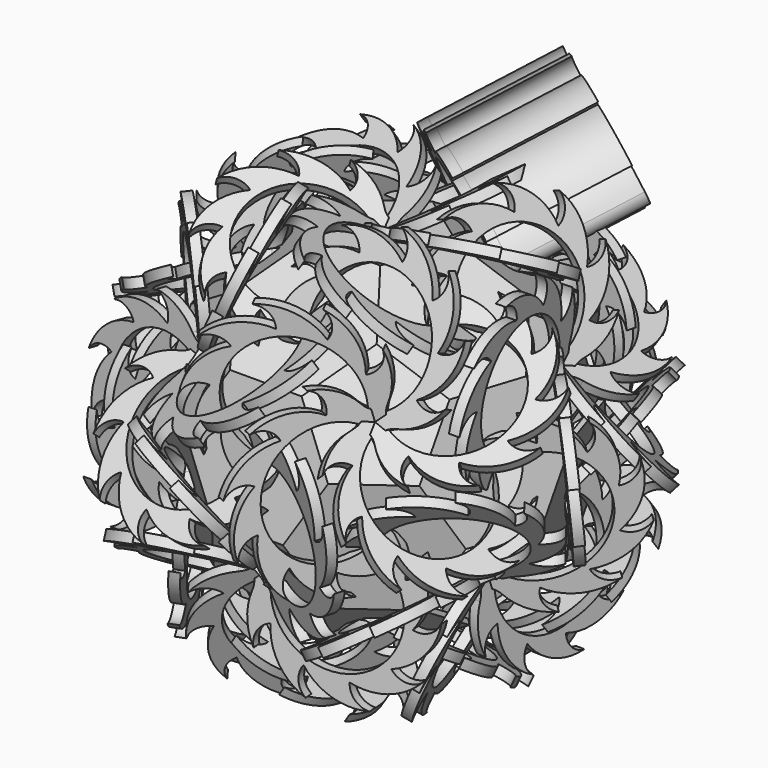
from build123d import *

# Parameters (mm, degrees)
F2_DEPTH  = 1
F3_DEPTH  = 1
F4_ANGLE  = -37.377368
F6_COUNT  = 5
F6_ANGLE  = 288
F9_DEPTH  = 2
F10_R     = 5
F12_ANGLE = 65
F13_COUNT = 5
F13_ANGLE = 288
F15_COUNT = 3
F15_ANGLE = 240
F16_COUNT = 5
F16_ANGLE = 288
F17_COUNT = 2
F17_ANGLE = 120
F18_COUNT = 3
F18_ANGLE = 240
F22_COUNT = 3
F22_ANGLE = 144
F26_COUNT = 3
F26_ANGLE = 144
F29_COUNT = 2
F29_ANGLE = 120
F32_COUNT = 3
F32_ANGLE = 144
F36_COUNT = 3
F36_ANGLE = 240
F40_COUNT = 3
F40_ANGLE = 144
F44_COUNT = 3
F44_ANGLE = 144
F48_COUNT = 2
F48_ANGLE = 120
F52_COUNT = 2
F52_ANGLE = 120
F56_COUNT = 2
F56_ANGLE = 120
F60_COUNT = 2
F60_ANGLE = 120
F66_DEPTH = 25


with BuildPart() as f2:
    # F0 (on Top) → F2 (new body)
    with BuildSketch(Plane.XY):
        Polygon((0, -10.3228644035), (7.5, -10.3228644035), (12.1352549156, 3.9429833409), (0, 12.7597621253), align=None)
        Polygon((-7.5, -10.3228644035), (0, -10.3228644035), (0, 12.7597621253), (-12.1352549156, 3.9429833409), align=None)
    extrude(amount=-F2_DEPTH)


with BuildPart() as f3:
    # F1 (on Top) → F3 (new body)
    with BuildSketch(Plane.XY):
        Polygon((32.2091731064, -18.3513614234), (36.844428022, -4.085513679), (26.8074689266, 7.0616587032), (12.1352549156, 3.9429833409), (7.5, -10.3228644035), (17.5369590954, -21.4700367857), align=None)
    extrude(amount=-F3_DEPTH)


with BuildPart() as f3_1:
    # F4: moved
    add(f3.part.rotate(Axis((9.8176274578, -3.1899405313, 0), (-0.3090169944, -0.9510565163, 0)), F4_ANGLE))


with BuildPart() as f6_1:
    # F6: instance of F3
    add(f3_1.part.rotate(Axis((0, 0, 3.8664315362), (0, 0, 1)), 1 * F6_ANGLE / (F6_COUNT - 1)))


with BuildPart() as f6_2:
    # F6: instance of F3
    add(f3_1.part.rotate(Axis((0, 0, 3.8664315362), (0, 0, 1)), 2 * F6_ANGLE / (F6_COUNT - 1)))


with BuildPart() as f6_3:
    # F6: instance of F3
    add(f3_1.part.rotate(Axis((0, 0, 3.8664315362), (0, 0, 1)), 3 * F6_ANGLE / (F6_COUNT - 1)))


with BuildPart() as f6_4:
    # F6: instance of F3
    add(f3_1.part.rotate(Axis((0, 0, 3.8664315362), (0, 0, 1)), 4 * F6_ANGLE / (F6_COUNT - 1)))


with BuildPart() as f9:
    # F8 (on Right) → F9 (new body)
    with BuildSketch(Plane.YZ):
        with BuildLine():
            ThreePointArc((-20.0381562793, -7.4218225341), (-18.0432138806, 14.7456768661), (-1.371596125, 0))
            ThreePointArc((-1.371596125, 0), (1.2710572909, -2.1110060804), (1.0658705895, 1.265065922))
            ThreePointArc((1.0658705895, 1.265065922), (3.462744203, 7.3677169674), (2.5001799222, 13.8531485572))
            ThreePointArc((2.5001799222, 13.8531485572), (1.8396441745, 10.7438611605), (-0.8004298525, 8.9735547684))
            ThreePointArc((-0.8004298525, 8.9735547684), (-2.1304901639, 15.9377846017), (-6.983453041, 21.1067602176))
            ThreePointArc((-6.983453041, 21.1067602176), (-5.7243130519, 18.2607184854), (-6.7542303289, 15.3239417734))
            ThreePointArc((-6.7542303289, 15.3239417734), (-11.923743314, 20.1763322255), (-18.8881203911, 21.5056213332))
            ThreePointArc((-18.8881203911, 21.5056213332), (-16.196593384, 19.9432291213), (-15.3036199233, 16.9619566661))
            ThreePointArc((-15.3036199233, 16.9619566661), (-22.3380073271, 17.8490595111), (-28.7536432712, 14.8309188523))
            ThreePointArc((-28.7536432712, 14.8309188523), (-25.6578010812, 15.1489568819), (-23.1830223937, 13.2619334316))
            ThreePointArc((-23.1830223937, 13.2619334316), (-29.3953873179, 9.8449055341), (-32.8117272579, 3.6321622578))
            ThreePointArc((-32.8117272579, 3.6321622578), (-30.4940763777, 5.7091508113), (-27.3827738075, 5.6371551864))
            ThreePointArc((-27.3827738075, 5.6371551864), (-30.4002040016, -0.7788149372), (-29.5123221974, -7.813104063))
            ThreePointArc((-29.5123221974, -7.813104063), (-28.8581264893, -4.7705040188), (-26.2987118688, -2.9999719366))
            ThreePointArc((-26.2987118688, -2.9999719366), (-26.0274642787, -7.0575500385), (-24.4889350399, -10.821914937))
            ThreePointArc((-24.4889350399, -10.821914937), (-20.5634994581, -11.3472581158), (-20.0381562793, -7.4218225341))
        make_face()
    extrude(amount=-F9_DEPTH)

    # F10
    f10_edges = [f9.edges().sort_by_distance(p)[0] for p in [
        (-1, 1.065871, 1.265066),
    ]]
    fillet(f10_edges, radius=F10_R)


with BuildPart() as f9_1:
    # F12: moved
    add(f9.part.rotate(Axis((0, -10.3228644132, -3.9429833282), (0, -0.9341723595, -0.3568220885)), F12_ANGLE))


with BuildPart() as f13_1:
    # F13: instance of F9
    add(f9_1.part.rotate(Axis((0, 0, 14.2103461549), (0, 0, 1)), 1 * F13_ANGLE / (F13_COUNT - 1)))


with BuildPart() as f13_2:
    # F13: instance of F9
    add(f9_1.part.rotate(Axis((0, 0, 14.2103461549), (0, 0, 1)), 2 * F13_ANGLE / (F13_COUNT - 1)))


with BuildPart() as f13_3:
    # F13: instance of F9
    add(f9_1.part.rotate(Axis((0, 0, 14.2103461549), (0, 0, 1)), 3 * F13_ANGLE / (F13_COUNT - 1)))


with BuildPart() as f13_4:
    # F13: instance of F9
    add(f9_1.part.rotate(Axis((0, 0, 14.2103461549), (0, 0, 1)), 4 * F13_ANGLE / (F13_COUNT - 1)))


with BuildPart() as f15_1:
    # F15: instance of F9
    add(f9_1.part.rotate(Axis((0, -25.3455492518, -1.7338218178), (0, -0.6070619963, 0.7946544738)), 1 * F15_ANGLE / (F15_COUNT - 1)))


with BuildPart() as f15_2:
    # F15: instance of F9
    add(f9_1.part.rotate(Axis((0, -25.3455492518, -1.7338218178), (0, -0.6070619963, 0.7946544738)), 2 * F15_ANGLE / (F15_COUNT - 1)))


with BuildPart() as f16_1:
    # F16: instance of F15_2
    add(f15_2.part.rotate(Axis((0, 0, 14.2103461549), (0, 0, 1)), 1 * F16_ANGLE / (F16_COUNT - 1)))


with BuildPart() as f16_2:
    # F16: instance of F15_2
    add(f15_2.part.rotate(Axis((0, 0, 14.2103461549), (0, 0, 1)), 2 * F16_ANGLE / (F16_COUNT - 1)))


with BuildPart() as f16_3:
    # F16: instance of F15_2
    add(f15_2.part.rotate(Axis((0, 0, 14.2103461549), (0, 0, 1)), 3 * F16_ANGLE / (F16_COUNT - 1)))


with BuildPart() as f16_4:
    # F16: instance of F15_2
    add(f15_2.part.rotate(Axis((0, 0, 14.2103461549), (0, 0, 1)), 4 * F16_ANGLE / (F16_COUNT - 1)))


with BuildPart() as f16_5:
    # F16: instance of F15_1
    add(f15_1.part.rotate(Axis((0, 0, 14.2103461549), (0, 0, 1)), 1 * F16_ANGLE / (F16_COUNT - 1)))


with BuildPart() as f16_6:
    # F16: instance of F15_1
    add(f15_1.part.rotate(Axis((0, 0, 14.2103461549), (0, 0, 1)), 2 * F16_ANGLE / (F16_COUNT - 1)))


with BuildPart() as f16_7:
    # F16: instance of F15_1
    add(f15_1.part.rotate(Axis((0, 0, 14.2103461549), (0, 0, 1)), 3 * F16_ANGLE / (F16_COUNT - 1)))


with BuildPart() as f16_8:
    # F16: instance of F15_1
    add(f15_1.part.rotate(Axis((0, 0, 14.2103461549), (0, 0, 1)), 4 * F16_ANGLE / (F16_COUNT - 1)))


with BuildPart() as f17_1:
    # F17: instance of F3
    add(f3_1.part.rotate(Axis((0, -25.3455492518, -1.7338218178), (0, 0.6070619963, -0.7946544738)), 1 * F17_ANGLE / (F17_COUNT - 1)))


with BuildPart() as f17_2:
    # F17: instance of F16_5
    add(f16_5.part.rotate(Axis((0, -25.3455492518, -1.7338218178), (0, 0.6070619963, -0.7946544738)), 1 * F17_ANGLE / (F17_COUNT - 1)))


with BuildPart() as f17_3:
    # F17: instance of F13_1
    add(f13_1.part.rotate(Axis((0, -25.3455492518, -1.7338218178), (0, 0.6070619963, -0.7946544738)), 1 * F17_ANGLE / (F17_COUNT - 1)))


with BuildPart() as f17_4:
    # F17: instance of F16_1
    add(f16_1.part.rotate(Axis((0, -25.3455492518, -1.7338218178), (0, 0.6070619963, -0.7946544738)), 1 * F17_ANGLE / (F17_COUNT - 1)))


with BuildPart() as f18_1:
    # F18: instance of F2
    add(f2.part.rotate(Axis((0, -25.3455492518, -1.7338218178), (0, -0.6070619963, 0.7946544738)), 1 * F18_ANGLE / (F18_COUNT - 1)))


with BuildPart() as f18_2:
    # F18: instance of F2
    add(f2.part.rotate(Axis((0, -25.3455492518, -1.7338218178), (0, -0.6070619963, 0.7946544738)), 2 * F18_ANGLE / (F18_COUNT - 1)))


with BuildPart() as f18_3:
    # F18: instance of F13_2
    add(f13_2.part.rotate(Axis((0, -25.3455492518, -1.7338218178), (0, -0.6070619963, 0.7946544738)), 1 * F18_ANGLE / (F18_COUNT - 1)))


with BuildPart() as f18_4:
    # F18: instance of F13_2
    add(f13_2.part.rotate(Axis((0, -25.3455492518, -1.7338218178), (0, -0.6070619963, 0.7946544738)), 2 * F18_ANGLE / (F18_COUNT - 1)))


with BuildPart() as f18_5:
    # F18: instance of F13_3
    add(f13_3.part.rotate(Axis((0, -25.3455492518, -1.7338218178), (0, -0.6070619963, 0.7946544738)), 1 * F18_ANGLE / (F18_COUNT - 1)))


with BuildPart() as f18_6:
    # F18: instance of F13_3
    add(f13_3.part.rotate(Axis((0, -25.3455492518, -1.7338218178), (0, -0.6070619963, 0.7946544738)), 2 * F18_ANGLE / (F18_COUNT - 1)))


with BuildPart() as f22_1:
    # F22: instance of F17_1
    add(f17_1.part.rotate(Axis((-18.9711930891, -26.1116072266, -18.7737157723), (0.5257311104, 0.7236067968, -0.4472135991)), 1 * F22_ANGLE / (F22_COUNT - 1)))


with BuildPart() as f22_2:
    # F22: instance of F17_1
    add(f17_1.part.rotate(Axis((-18.9711930891, -26.1116072266, -18.7737157723), (0.5257311104, 0.7236067968, -0.4472135991)), 2 * F22_ANGLE / (F22_COUNT - 1)))


with BuildPart() as f22_3:
    # F22: instance of F17_3
    add(f17_3.part.rotate(Axis((-18.9711930891, -26.1116072266, -18.7737157723), (0.5257311104, 0.7236067968, -0.4472135991)), 1 * F22_ANGLE / (F22_COUNT - 1)))


with BuildPart() as f22_4:
    # F22: instance of F17_3
    add(f17_3.part.rotate(Axis((-18.9711930891, -26.1116072266, -18.7737157723), (0.5257311104, 0.7236067968, -0.4472135991)), 2 * F22_ANGLE / (F22_COUNT - 1)))


with BuildPart() as f22_5:
    # F22: instance of F17_4
    add(f17_4.part.rotate(Axis((-18.9711930891, -26.1116072266, -18.7737157723), (0.5257311104, 0.7236067968, -0.4472135991)), 1 * F22_ANGLE / (F22_COUNT - 1)))


with BuildPart() as f22_6:
    # F22: instance of F17_4
    add(f17_4.part.rotate(Axis((-18.9711930891, -26.1116072266, -18.7737157723), (0.5257311104, 0.7236067968, -0.4472135991)), 2 * F22_ANGLE / (F22_COUNT - 1)))


with BuildPart() as f22_7:
    # F22: instance of F17_2
    add(f17_2.part.rotate(Axis((-18.9711930891, -26.1116072266, -18.7737157723), (0.5257311104, 0.7236067968, -0.4472135991)), 1 * F22_ANGLE / (F22_COUNT - 1)))


with BuildPart() as f22_8:
    # F22: instance of F17_2
    add(f17_2.part.rotate(Axis((-18.9711930891, -26.1116072266, -18.7737157723), (0.5257311104, 0.7236067968, -0.4472135991)), 2 * F22_ANGLE / (F22_COUNT - 1)))


with BuildPart() as f26_1:
    # F26: instance of F3
    add(f3_1.part.rotate(Axis((20.2758098134, -27.9072581024, -17.6639424888), (-0.5257311104, 0.7236067968, -0.4472135991)), 1 * F26_ANGLE / (F26_COUNT - 1)))


with BuildPart() as f26_2:
    # F26: instance of F3
    add(f3_1.part.rotate(Axis((20.2758098134, -27.9072581024, -17.6639424888), (-0.5257311104, 0.7236067968, -0.4472135991)), 2 * F26_ANGLE / (F26_COUNT - 1)))


with BuildPart() as f26_3:
    # F26: instance of F16_1
    add(f16_1.part.rotate(Axis((20.2758098134, -27.9072581024, -17.6639424888), (-0.5257311104, 0.7236067968, -0.4472135991)), 1 * F26_ANGLE / (F26_COUNT - 1)))


with BuildPart() as f26_4:
    # F26: instance of F16_1
    add(f16_1.part.rotate(Axis((20.2758098134, -27.9072581024, -17.6639424888), (-0.5257311104, 0.7236067968, -0.4472135991)), 2 * F26_ANGLE / (F26_COUNT - 1)))


with BuildPart() as f26_5:
    # F26: instance of F13_1
    add(f13_1.part.rotate(Axis((20.2758098134, -27.9072581024, -17.6639424888), (-0.5257311104, 0.7236067968, -0.4472135991)), 1 * F26_ANGLE / (F26_COUNT - 1)))


with BuildPart() as f26_6:
    # F26: instance of F13_1
    add(f13_1.part.rotate(Axis((20.2758098134, -27.9072581024, -17.6639424888), (-0.5257311104, 0.7236067968, -0.4472135991)), 2 * F26_ANGLE / (F26_COUNT - 1)))


with BuildPart() as f26_7:
    # F26: instance of F16_5
    add(f16_5.part.rotate(Axis((20.2758098134, -27.9072581024, -17.6639424888), (-0.5257311104, 0.7236067968, -0.4472135991)), 1 * F26_ANGLE / (F26_COUNT - 1)))


with BuildPart() as f26_8:
    # F26: instance of F16_5
    add(f16_5.part.rotate(Axis((20.2758098134, -27.9072581024, -17.6639424888), (-0.5257311104, 0.7236067968, -0.4472135991)), 2 * F26_ANGLE / (F26_COUNT - 1)))


with BuildPart() as f29_1:
    # F29: instance of F18_2
    add(f18_2.part.rotate(Axis((0, -40.5030693029, -27.1761785704), (0, 0.9822469455, -0.1875924789)), 1 * F29_ANGLE / (F29_COUNT - 1)))


with BuildPart() as f32_1:
    # F32: instance of F26_2
    add(f26_2.part.rotate(Axis((0, -41.1465715097, -55.4848620892), (0, 0.8944271941, 0.4472135893)), 1 * F32_ANGLE / (F32_COUNT - 1)))


with BuildPart() as f32_2:
    # F32: instance of F26_2
    add(f26_2.part.rotate(Axis((0, -41.1465715097, -55.4848620892), (0, 0.8944271941, 0.4472135893)), 2 * F32_ANGLE / (F32_COUNT - 1)))


with BuildPart() as f32_3:
    # F32: instance of F26_4
    add(f26_4.part.rotate(Axis((0, -41.1465715097, -55.4848620892), (0, 0.8944271941, 0.4472135893)), 1 * F32_ANGLE / (F32_COUNT - 1)))


with BuildPart() as f32_4:
    # F32: instance of F26_4
    add(f26_4.part.rotate(Axis((0, -41.1465715097, -55.4848620892), (0, 0.8944271941, 0.4472135893)), 2 * F32_ANGLE / (F32_COUNT - 1)))


with BuildPart() as f32_5:
    # F32: instance of F26_6
    add(f26_6.part.rotate(Axis((0, -41.1465715097, -55.4848620892), (0, 0.8944271941, 0.4472135893)), 1 * F32_ANGLE / (F32_COUNT - 1)))


with BuildPart() as f32_6:
    # F32: instance of F26_6
    add(f26_6.part.rotate(Axis((0, -41.1465715097, -55.4848620892), (0, 0.8944271941, 0.4472135893)), 2 * F32_ANGLE / (F32_COUNT - 1)))


with BuildPart() as f32_7:
    # F32: instance of F18_4
    add(f18_4.part.rotate(Axis((0, -41.1465715097, -55.4848620892), (0, 0.8944271941, 0.4472135893)), 1 * F32_ANGLE / (F32_COUNT - 1)))


with BuildPart() as f32_8:
    # F32: instance of F18_4
    add(f18_4.part.rotate(Axis((0, -41.1465715097, -55.4848620892), (0, 0.8944271941, 0.4472135893)), 2 * F32_ANGLE / (F32_COUNT - 1)))


with BuildPart() as f36_1:
    # F36: instance of F2
    add(f2.part.rotate(Axis((-17.4030966331, 23.953307566, 3.8456892929), (0.3568220886, -0.4911234716, -0.7946544738)), 1 * F36_ANGLE / (F36_COUNT - 1)))


with BuildPart() as f36_2:
    # F36: instance of F2
    add(f2.part.rotate(Axis((-17.4030966331, 23.953307566, 3.8456892929), (0.3568220886, -0.4911234716, -0.7946544738)), 2 * F36_ANGLE / (F36_COUNT - 1)))


with BuildPart() as f40_1:
    # F40: instance of F22_2
    add(f22_2.part.rotate(Axis((-43.9943598437, 14.2946340797, -11.7823727251), (0.8506508064, -0.2763932025, -0.4472135991)), 1 * F40_ANGLE / (F40_COUNT - 1)))


with BuildPart() as f40_2:
    # F40: instance of F22_2
    add(f22_2.part.rotate(Axis((-43.9943598437, 14.2946340797, -11.7823727251), (0.8506508064, -0.2763932025, -0.4472135991)), 2 * F40_ANGLE / (F40_COUNT - 1)))


with BuildPart() as f40_3:
    # F40: instance of F22_6
    add(f22_6.part.rotate(Axis((-43.9943598437, 14.2946340797, -11.7823727251), (0.8506508064, -0.2763932025, -0.4472135991)), 1 * F40_ANGLE / (F40_COUNT - 1)))


with BuildPart() as f40_4:
    # F40: instance of F22_6
    add(f22_6.part.rotate(Axis((-43.9943598437, 14.2946340797, -11.7823727251), (0.8506508064, -0.2763932025, -0.4472135991)), 2 * F40_ANGLE / (F40_COUNT - 1)))


with BuildPart() as f40_5:
    # F40: instance of F22_4
    add(f22_4.part.rotate(Axis((-43.9943598437, 14.2946340797, -11.7823727251), (0.8506508064, -0.2763932025, -0.4472135991)), 1 * F40_ANGLE / (F40_COUNT - 1)))


with BuildPart() as f40_6:
    # F40: instance of F22_4
    add(f22_4.part.rotate(Axis((-43.9943598437, 14.2946340797, -11.7823727251), (0.8506508064, -0.2763932025, -0.4472135991)), 2 * F40_ANGLE / (F40_COUNT - 1)))


with BuildPart() as f40_7:
    # F40: instance of F18_3
    add(f18_3.part.rotate(Axis((-43.9943598437, 14.2946340797, -11.7823727251), (0.8506508064, -0.2763932025, -0.4472135991)), 1 * F40_ANGLE / (F40_COUNT - 1)))


with BuildPart() as f40_8:
    # F40: instance of F18_3
    add(f18_3.part.rotate(Axis((-43.9943598437, 14.2946340797, -11.7823727251), (0.8506508064, -0.2763932025, -0.4472135991)), 2 * F40_ANGLE / (F40_COUNT - 1)))


with BuildPart() as f44_1:
    # F44: instance of F40_2
    add(f40_2.part.rotate(Axis((1.534e-07, 54.8190866503, -7.5020330917), (-6.9e-09, -0.8944271892, -0.4472135991)), 1 * F44_ANGLE / (F44_COUNT - 1)))


with BuildPart() as f44_2:
    # F44: instance of F40_2
    add(f40_2.part.rotate(Axis((1.534e-07, 54.8190866503, -7.5020330917), (-6.9e-09, -0.8944271892, -0.4472135991)), 2 * F44_ANGLE / (F44_COUNT - 1)))


with BuildPart() as f44_3:
    # F44: instance of F40_6
    add(f40_6.part.rotate(Axis((1.534e-07, 54.8190866503, -7.5020330917), (-6.9e-09, -0.8944271892, -0.4472135991)), 1 * F44_ANGLE / (F44_COUNT - 1)))


with BuildPart() as f44_4:
    # F44: instance of F40_6
    add(f40_6.part.rotate(Axis((1.534e-07, 54.8190866503, -7.5020330917), (-6.9e-09, -0.8944271892, -0.4472135991)), 2 * F44_ANGLE / (F44_COUNT - 1)))


with BuildPart() as f44_5:
    # F44: instance of F40_8
    add(f40_8.part.rotate(Axis((1.534e-07, 54.8190866503, -7.5020330917), (-6.9e-09, -0.8944271892, -0.4472135991)), 1 * F44_ANGLE / (F44_COUNT - 1)))


with BuildPart() as f44_6:
    # F44: instance of F40_8
    add(f40_8.part.rotate(Axis((1.534e-07, 54.8190866503, -7.5020330917), (-6.9e-09, -0.8944271892, -0.4472135991)), 2 * F44_ANGLE / (F44_COUNT - 1)))


with BuildPart() as f44_7:
    # F44: instance of F40_4
    add(f40_4.part.rotate(Axis((1.534e-07, 54.8190866503, -7.5020330917), (-6.9e-09, -0.8944271892, -0.4472135991)), 1 * F44_ANGLE / (F44_COUNT - 1)))


with BuildPart() as f44_8:
    # F44: instance of F40_4
    add(f40_4.part.rotate(Axis((1.534e-07, 54.8190866503, -7.5020330917), (-6.9e-09, -0.8944271892, -0.4472135991)), 2 * F44_ANGLE / (F44_COUNT - 1)))


with BuildPart() as f48_1:
    # F48: instance of F22_2
    add(f22_2.part.rotate(Axis((-45.320051719, 14.7253777202, -44.0123603845), (0.9341723533, -0.3035310175, 0.1875924726)), 1 * F48_ANGLE / (F48_COUNT - 1)))


with BuildPart() as f48_2:
    # F48: instance of F22_4
    add(f22_4.part.rotate(Axis((-45.320051719, 14.7253777202, -44.0123603845), (0.9341723533, -0.3035310175, 0.1875924726)), 1 * F48_ANGLE / (F48_COUNT - 1)))


with BuildPart() as f48_3:
    # F48: instance of F22_6
    add(f22_6.part.rotate(Axis((-45.320051719, 14.7253777202, -44.0123603845), (0.9341723533, -0.3035310175, 0.1875924726)), 1 * F48_ANGLE / (F48_COUNT - 1)))


with BuildPart() as f48_4:
    # F48: instance of F18_3
    add(f18_3.part.rotate(Axis((-45.320051719, 14.7253777202, -44.0123603845), (0.9341723533, -0.3035310175, 0.1875924726)), 1 * F48_ANGLE / (F48_COUNT - 1)))


with BuildPart() as f52_1:
    # F52: instance of F16_5
    add(f16_5.part.rotate(Axis((51.1630279448, -16.6238756598, -24.6374564773), (-0.9341723577, 0.3035310035, -0.1875924733)), 1 * F52_ANGLE / (F52_COUNT - 1)))


with BuildPart() as f52_2:
    # F52: instance of F13_1
    add(f13_1.part.rotate(Axis((51.1630279448, -16.6238756598, -24.6374564773), (-0.9341723577, 0.3035310035, -0.1875924733)), 1 * F52_ANGLE / (F52_COUNT - 1)))


with BuildPart() as f52_3:
    # F52: instance of F16_1
    add(f16_1.part.rotate(Axis((51.1630279448, -16.6238756598, -24.6374564773), (-0.9341723577, 0.3035310035, -0.1875924733)), 1 * F52_ANGLE / (F52_COUNT - 1)))


with BuildPart() as f52_4:
    # F52: instance of F3
    add(f3_1.part.rotate(Axis((51.1630279448, -16.6238756598, -24.6374564773), (-0.9341723577, 0.3035310035, -0.1875924733)), 1 * F52_ANGLE / (F52_COUNT - 1)))


with BuildPart() as f56_1:
    # F56: instance of F26_2
    add(f26_2.part.rotate(Axis((20.2389789509, -27.8565650407, -79.9844450272), (-0.3568220897, 0.4911234788, 0.7946544689)), 1 * F56_ANGLE / (F56_COUNT - 1)))


with BuildPart() as f56_2:
    # F56: instance of F26_4
    add(f26_4.part.rotate(Axis((20.2389789509, -27.8565650407, -79.9844450272), (-0.3568220897, 0.4911234788, 0.7946544689)), 1 * F56_ANGLE / (F56_COUNT - 1)))


with BuildPart() as f56_3:
    # F56: instance of F26_6
    add(f26_6.part.rotate(Axis((20.2389789509, -27.8565650407, -79.9844450272), (-0.3568220897, 0.4911234788, 0.7946544689)), 1 * F56_ANGLE / (F56_COUNT - 1)))


with BuildPart() as f56_4:
    # F56: instance of F18_4
    add(f18_4.part.rotate(Axis((20.2389789509, -27.8565650407, -79.9844450272), (-0.3568220897, 0.4911234788, 0.7946544689)), 1 * F56_ANGLE / (F56_COUNT - 1)))


with BuildPart() as f60_1:
    # F60: instance of F52_4
    add(f52_4.part.rotate(Axis((24.2012826257, 7.8634731584, -68.221784607), (-0.5773502692, -0.1875924683, 0.7946544737)), 1 * F60_ANGLE / (F60_COUNT - 1)))


with BuildPart() as f60_2:
    # F60: instance of F52_3
    add(f52_3.part.rotate(Axis((24.2012826257, 7.8634731584, -68.221784607), (-0.5773502692, -0.1875924683, 0.7946544737)), 1 * F60_ANGLE / (F60_COUNT - 1)))


with BuildPart() as f60_3:
    # F60: instance of F52_1
    add(f52_1.part.rotate(Axis((24.2012826257, 7.8634731584, -68.221784607), (-0.5773502692, -0.1875924683, 0.7946544737)), 1 * F60_ANGLE / (F60_COUNT - 1)))


with BuildPart() as f60_4:
    # F60: instance of F52_2
    add(f52_2.part.rotate(Axis((24.2012826257, 7.8634731584, -68.221784607), (-0.5773502692, -0.1875924683, 0.7946544737)), 1 * F60_ANGLE / (F60_COUNT - 1)))


with BuildPart() as f66:
    # F66 (new): a face of the model
    f66_faces = [f16_2.part.faces().sort_by_distance(p)[0] for p in [
        (1.31810176, 30.9628284564, -20.5883774051),
    ]]
    extrude(f66_faces, amount=F66_DEPTH)


solid = Compound([f2.part, f3_1.part, f6_1.part, f6_2.part, f6_3.part, f6_4.part, f9_1.part, f13_1.part, f13_2.part, f13_3.part, f13_4.part, f15_1.part, f15_2.part, f16_1.part, f16_2.part, f16_3.part, f16_4.part, f16_5.part, f16_6.part, f16_7.part, f16_8.part, f17_1.part, f17_2.part, f17_3.part, f17_4.part, f18_1.part, f18_2.part, f18_3.part, f18_4.part, f18_5.part, f18_6.part, f22_1.part, f22_2.part, f22_3.part, f22_4.part, f22_5.part, f22_6.part, f26_1.part, f26_2.part, f26_3.part, f26_4.part, f26_5.part, f26_6.part, f29_1.part, f32_1.part, f32_2.part, f32_3.part, f32_4.part, f32_5.part, f32_6.part, f32_7.part, f32_8.part, f36_1.part, f36_2.part, f40_1.part, f40_2.part, f40_3.part, f40_4.part, f40_5.part, f40_6.part, f40_7.part, f40_8.part, f44_1.part, f44_2.part, f44_3.part, f44_4.part, f44_5.part, f44_6.part, f44_7.part, f44_8.part, f48_1.part, f48_2.part, f48_3.part, f48_4.part, f52_1.part, f52_2.part, f52_3.part, f52_4.part, f56_1.part, f56_2.part, f56_3.part, f56_4.part, f60_1.part, f60_2.part, f60_3.part, f60_4.part, f66.part])
